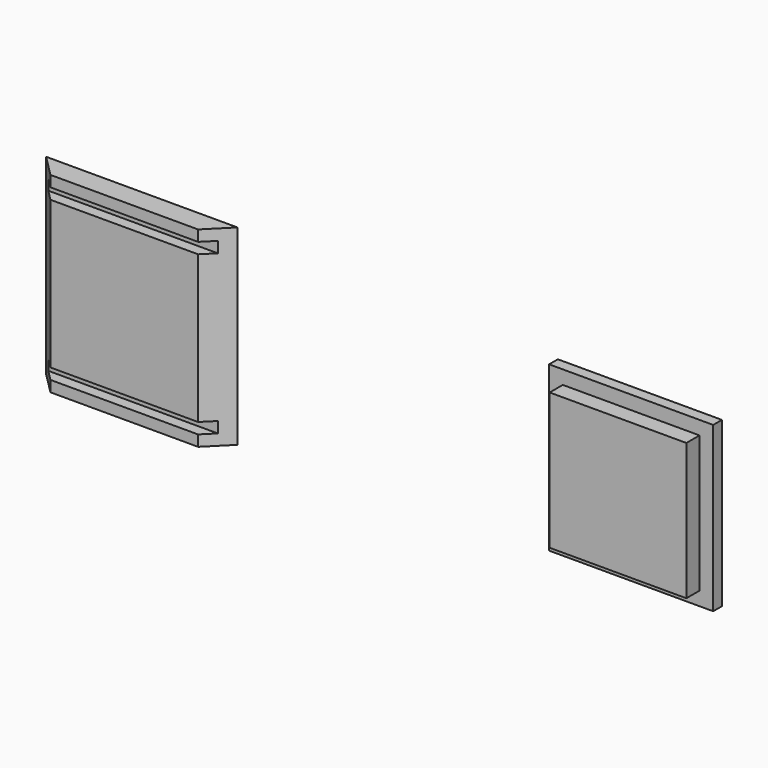
from build123d import *

# Parameters (mm, degrees)
F0_W     = 70
F0_H     = 70
F1_DEPTH = 8
F2_W     = 70
F2_H     = 4
F3_DEPTH = 4
F4_SIZE  = 7.99999
F5_W     = 60
F5_H     = 60
F6_DEPTH = 10
F7_W     = 60
F7_H     = 60
F7_W_2   = 50
F7_H_2   = 50
F8_DEPTH = 6


# Not quite as in the source:
# - a fillet or chamfer is up to 0.001 mm smaller than in the source, because OpenCascade refuses the exact size


with BuildPart() as f1:
    # F0 (on Front) → F1 (new body)
    with BuildSketch(Plane.XZ):
        with Locations((-1024.4680345058, -62.2741735576)):
            Rectangle(F0_W, F0_H)
    extrude(amount=F1_DEPTH)

    # F2 (on face) → F3 (cut)
    with BuildSketch(Plane.XZ.offset(8)):
        with Locations((-1024.4680345058, -33.2741735576)):
            Rectangle(F2_W, F2_H)
        with Locations((-1024.4680345058, -91.2741735576)):
            Rectangle(F2_W, F2_H)
    extrude(amount=-F3_DEPTH, mode=Mode.SUBTRACT)

    # F4 (size 8 in the source; OpenCascade refuses exactly that, so slightly less here)
    f4_edges = [f1.edges().sort_by_distance(p)[0] for p in [
        (-989.468035, -8, -62.274174),
        (-1059.468035, -8, -62.274174),
    ]]
    chamfer(f4_edges, length=F4_SIZE)


with BuildPart() as f6:
    # F5 (on Front) → F6 (new body)
    with BuildSketch(Plane.XZ):
        with Locations((-842.2881662846, -61.6157978558)):
            Rectangle(F5_W, F5_H)
    extrude(amount=F6_DEPTH)

    # F7 (on face) → F8 (cut)
    with BuildSketch(Plane.XZ.offset(10)):
        with Locations((-842.2881662846, -61.6157978558)):
            Rectangle(F7_W, F7_H)
        with Locations((-842.2881662846, -61.6157978558)):
            Rectangle(F7_W_2, F7_H_2, mode=Mode.SUBTRACT)
    extrude(amount=-F8_DEPTH, mode=Mode.SUBTRACT)


solid = Compound([f1.part, f6.part])
